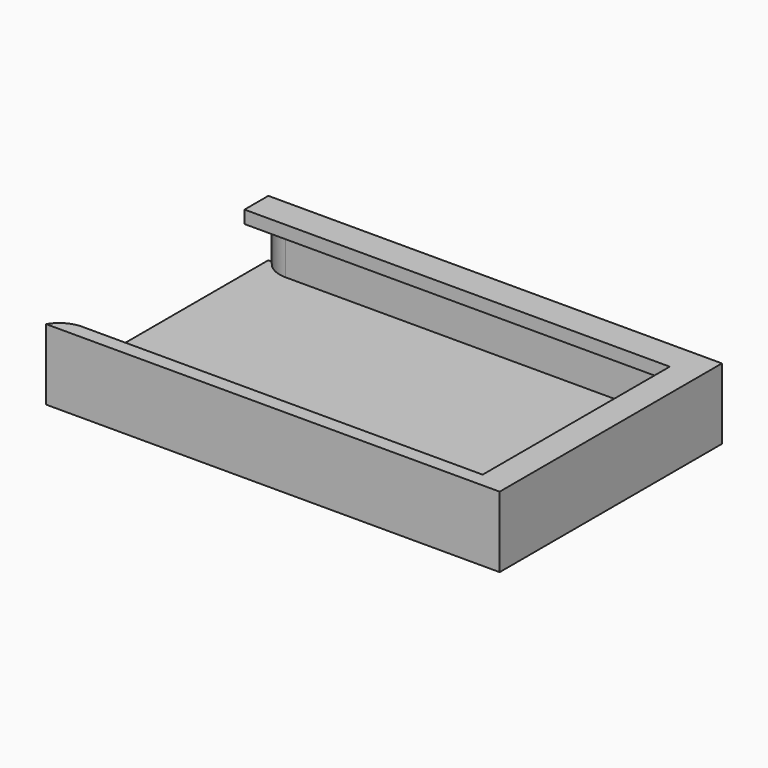
from build123d import *

# Parameters (mm, degrees)
F0_W        = 155
F0_H        = 88
F1_DEPTH    = 5
F0_W_2      = 5
F2_DEPTH    = 25
F3_W        = 155
F3_H        = 4.5
F4_DEPTH    = 5.5
F5_W        = 82.5
F5_H        = 4.5
F6_DEPTH    = 5
F7_T1_DEPTH = 41.6506350946
F7_T3_DEPTH = 15.5


# Not quite as in the source:
# - a fillet or chamfer that OpenCascade refuses, or shapes differently, is made with other operations: its cross-section is extruded or revolved along the edge and cut away or added


with BuildPart() as f1:
    # F0 (on Top) → F1 (new body)
    with BuildSketch(Plane.XY):
        with Locations((-2.5, 0)):
            Rectangle(F0_W, F0_H)
    extrude(amount=F1_DEPTH)

    # F0 (on Top) → F2 (join)
    with BuildSketch(Plane.XY):
        Polygon((75, 44), (80, 44), (80, 49), (-80, 49), (-80, 44), align=None)
        with Locations((77.5, 0)):
            Rectangle(F0_W_2, F0_H)
        Polygon((80, -49), (80, -44), (75, -44), (-80, -44), (-80, -49), align=None)
    extrude(amount=F2_DEPTH)

    # F3 (on face) → F4 (join)
    with BuildSketch(Plane.XZ.offset(-44)):
        with Locations((-2.5, 22.75)):
            Rectangle(F3_W, F3_H)
    extrude(amount=F4_DEPTH)

    # F5 (on face) → F6 (join)
    with BuildSketch(Plane(origin=(75, 0, 0), x_dir=(0, -1, 0), z_dir=(-1, 0, 0))):
        with Locations((2.75, 22.75)):
            Rectangle(F5_W, F5_H)
    extrude(amount=F6_DEPTH)

    # F7: fillet of radius 10 on 2 edges, made by hand

    # F7_s2 → F7_t1 (cut)
    with BuildSketch(Plane.XY.offset(5)):
        with BuildLine():
            ThreePointArc((-80, -49), (-76.3397459622, -45.3397459622), (-71.3397459622, -44))
            Line((-71.3397459622, -44), (-80, -44))
            Line((-80, -44), (-80, -49))
        make_face()
    extrude(amount=F7_T1_DEPTH, mode=Mode.SUBTRACT)

    # F7_s4 → F7_t3 (cut)
    with BuildSketch(Plane.XY.offset(5)):
        with BuildLine():
            ThreePointArc((-80, 54), (-77.0710678119, 46.9289321881), (-70, 44))
            Line((-70, 44), (-80, 44))
            Line((-80, 44), (-80, 54))
        make_face()
    extrude(amount=F7_T3_DEPTH, mode=Mode.SUBTRACT)


solid = f1.part
